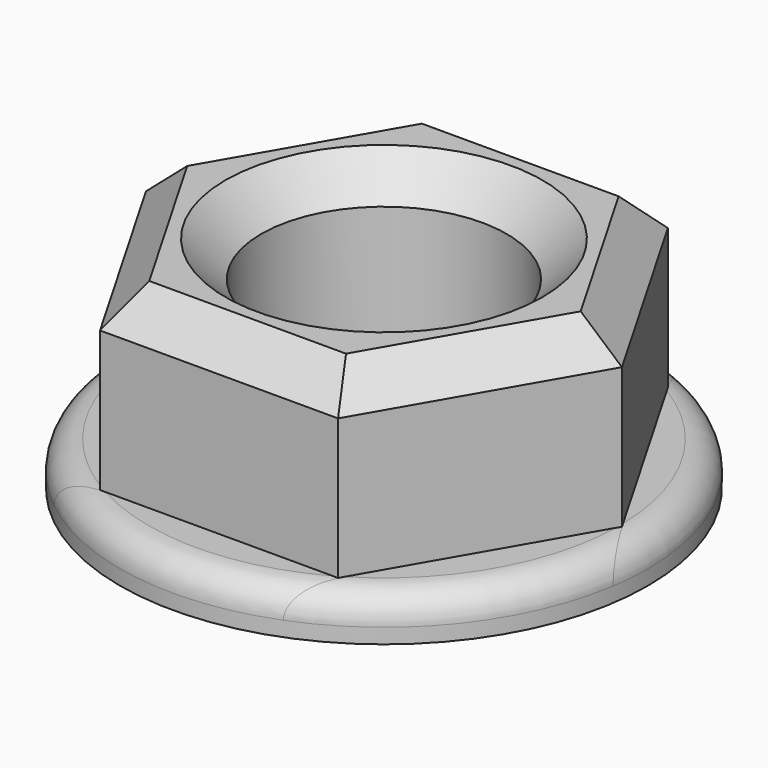
from build123d import *

# Parameters (mm, degrees)
F1_DEPTH = 7.8105
F0_R     = 9.37895
F2_DEPTH = 1.5494
F4_D     = 8.7249
F5_SIZE  = 1.27


# Not quite as in the source:
# - a fillet or chamfer that OpenCascade refuses, or shapes differently, is made with other operations: its cross-section is extruded or revolved along the edge and cut away or added


with BuildPart() as f1:
    # F0 (on Top) → F1 (new body)
    with BuildSketch(Plane.XY):
        Polygon((4.2291, 7.3250160703), (-4.2291, 7.3250160703), (-8.4582, 0), (-4.2291, -7.3250160703), (4.2291, -7.3250160703), (8.4582, 0), align=None)
    extrude(amount=F1_DEPTH)

    # F0 (on Top) → F2 (join)
    with BuildSketch(Plane.XY):
        Circle(F0_R)
        Polygon((-8.4582, 0), (-4.2291, 7.3250160703), (4.2291, 7.3250160703), (8.4582, 0), (4.2291, -7.3250160703), (-4.2291, -7.3250160703), align=None, mode=Mode.SUBTRACT)
    extrude(amount=F2_DEPTH)

    # F3: fillet of radius 1.016 on 1 edges, made by hand


with BuildPart() as f3_tool2:
    # F3_s3 → F3_t4 (revolve)
    with BuildSketch(Plane.XZ):
        with BuildLine():
            ThreePointArc((8.36295, 1.5494), (9.0813704897, 1.2518204897), (9.37895, 0.5334))
            Line((9.37895, 0.5334), (9.37895, 1.5494))
            Line((9.37895, 1.5494), (8.36295, 1.5494))
        make_face()
    revolve(axis=Axis((0, 0, 1.5494), (0, 0, 1)))

    split(bisect_by=Plane(origin=(6.34365, 3.6625080351, 0), x_dir=(0, 0, 1), z_dir=(0.8660254038, 0.5, 0)), keep=Keep.TOP)


with BuildPart() as f1_1:
    add(f1.part)

    # F3_t1: cut F3_tool2
    add(f3_tool2.part, mode=Mode.SUBTRACT)


with BuildPart() as f3_tool7:
    # F3_s8 → F3_t9 (revolve)
    with BuildSketch(Plane.XZ):
        with BuildLine():
            ThreePointArc((8.36295, 1.5494), (9.0813704897, 1.2518204897), (9.37895, 0.5334))
            Line((9.37895, 0.5334), (9.37895, 1.5494))
            Line((9.37895, 1.5494), (8.36295, 1.5494))
        make_face()
    revolve(axis=Axis((0, 0, 1.5494), (0, 0, 1)))

    split(bisect_by=Plane(origin=(6.34365, -3.6625080351, 0), x_dir=(0, 0, 1), z_dir=(0.8660254038, -0.5, 0)), keep=Keep.TOP)


with BuildPart() as f1_2:
    add(f1_1.part)

    # F3_t6: cut F3_tool7
    add(f3_tool7.part, mode=Mode.SUBTRACT)


with BuildPart() as f3_tool12:
    # F3_s13 → F3_t14 (revolve)
    with BuildSketch(Plane.XZ):
        with BuildLine():
            ThreePointArc((8.36295, 1.5494), (9.0813704897, 1.2518204897), (9.37895, 0.5334))
            Line((9.37895, 0.5334), (9.37895, 1.5494))
            Line((9.37895, 1.5494), (8.36295, 1.5494))
        make_face()
    revolve(axis=Axis((0, 0, 1.5494), (0, 0, 1)))

    split(bisect_by=Plane.XZ.offset(-7.3250160703), keep=Keep.BOTTOM)


with BuildPart() as f1_3:
    add(f1_2.part)

    # F3_t11: cut F3_tool12
    add(f3_tool12.part, mode=Mode.SUBTRACT)


with BuildPart() as f3_tool17:
    # F3_s18 → F3_t19 (revolve)
    with BuildSketch(Plane.XZ):
        with BuildLine():
            ThreePointArc((8.36295, 1.5494), (9.0813704897, 1.2518204897), (9.37895, 0.5334))
            Line((9.37895, 0.5334), (9.37895, 1.5494))
            Line((9.37895, 1.5494), (8.36295, 1.5494))
        make_face()
    revolve(axis=Axis((0, 0, 1.5494), (0, 0, 1)))

    split(bisect_by=Plane.XZ.offset(7.3250160703), keep=Keep.TOP)


with BuildPart() as f1_4:
    add(f1_3.part)

    # F3_t16: cut F3_tool17
    add(f3_tool17.part, mode=Mode.SUBTRACT)


with BuildPart() as f3_tool22:
    # F3_s23 → F3_t24 (revolve)
    with BuildSketch(Plane.XZ):
        with BuildLine():
            ThreePointArc((8.36295, 1.5494), (9.0813704897, 1.2518204897), (9.37895, 0.5334))
            Line((9.37895, 0.5334), (9.37895, 1.5494))
            Line((9.37895, 1.5494), (8.36295, 1.5494))
        make_face()
    revolve(axis=Axis((0, 0, 1.5494), (0, 0, 1)))

    split(bisect_by=Plane(origin=(-6.34365, 3.6625080351, 0), x_dir=(0, 0, 1), z_dir=(-0.8660254038, 0.5, 0)), keep=Keep.TOP)


with BuildPart() as f1_5:
    add(f1_4.part)

    # F3_t21: cut F3_tool22
    add(f3_tool22.part, mode=Mode.SUBTRACT)


with BuildPart() as f3_tool27:
    # F3_s28 → F3_t29 (revolve)
    with BuildSketch(Plane.XZ):
        with BuildLine():
            ThreePointArc((8.36295, 1.5494), (9.0813704897, 1.2518204897), (9.37895, 0.5334))
            Line((9.37895, 0.5334), (9.37895, 1.5494))
            Line((9.37895, 1.5494), (8.36295, 1.5494))
        make_face()
    revolve(axis=Axis((0, 0, 1.5494), (0, 0, 1)))

    split(bisect_by=Plane(origin=(-6.34365, -3.6625080351, 0), x_dir=(0, 0, 1), z_dir=(-0.8660254038, -0.5, 0)), keep=Keep.TOP)


with BuildPart() as f1_6:
    add(f1_5.part)

    # F3_t26: cut F3_tool27
    add(f3_tool27.part, mode=Mode.SUBTRACT)

    # F4 (through all)
    with Locations(Plane(origin=(0, 0, 0), x_dir=(1, 0, 0), z_dir=(0, 0, -1))):
        with Locations((0, 0)):
            Hole(F4_D / 2)

    # F5
    f5_edges = [f1_6.edges().sort_by_distance(p)[0] for p in [
        (0, 7.325016, 7.8105),
        (6.34365, 3.662508, 7.8105),
        (6.34365, -3.662508, 7.8105),
        (0, -7.325016, 7.8105),
        (-6.34365, -3.662508, 7.8105),
        (-6.34365, 3.662508, 7.8105),
        (-4.36245, 0, 7.8105),
        (-4.36245, 0, 0),
    ]]
    chamfer(f5_edges, length=F5_SIZE)


solid = f1_6.part
